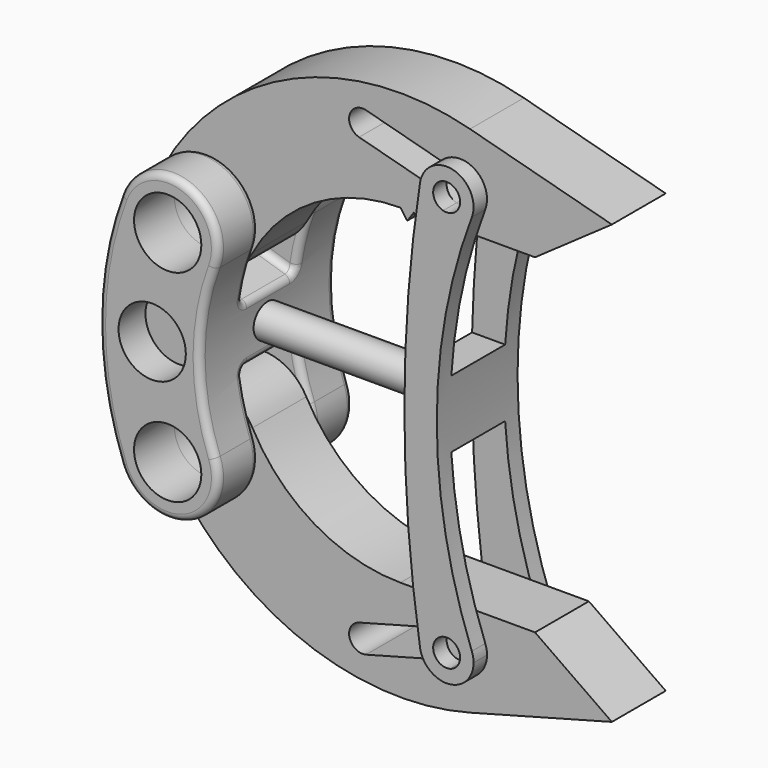
from build123d import *

# Parameters (mm, degrees)
F1_R           = 5
F2_DEPTH       = 5
F0_R           = 5
F3_DEPTH       = 12.5
F4_R           = 5
F5_DEPTH       = 25.001
F6_R           = 5
F7_DEPTH       = 5
F8_R           = 5
F9_DEPTH       = 7.5
F10_R          = 2.5
F11_DEPTH      = 10.2360656985
F11_DEPTH_BACK = 60.001
F12_R          = 2.5
F13_DEPTH      = 32
F13_DEPTH_BACK = 10
F15_DEPTH      = 7.5
F17_DEPTH      = 5
F18_R          = 1


with BuildPart() as f2:
    # F1 (on Front) → F2 (new body, symmetric)
    with BuildSketch(Plane.XZ):
        with BuildLine():
            ThreePointArc((38.9229935461, 38.1714845638), (12.7620087728, 36.2695311392), (-6.5959822677, 18.5697363943))
            ThreePointArc((-6.5959822677, 18.5697363943), (-3.5697363943, 8.4040177323), (6.5959822677, 11.4302636057))
            ThreePointArc((6.5959822677, 11.4302636057), (15.785676778, 21.0076181762), (28.5825898266, 24.5311422915))
            Line((28.5825898266, 24.5311422915), (30.5825898266, 24.5311422915))
            Line((30.5825898266, 24.5311422915), (32.5825898266, 24.5311422915))
            Line((32.5825898266, 24.5311422915), (48.5825898266, 24.5311422915))
            Line((48.5825898266, 24.5311422915), (60, 32.5311422915))
            Line((60, 32.5311422915), (38.9229935461, 38.1714845638))
        make_face()
        with Locations((0, 15)):
            Circle(F1_R, mode=Mode.SUBTRACT)
        with BuildLine():
            ThreePointArc((22.4425128865, 31.74578129), (21.0275159589, 34.1948185896), (23.4765532585, 35.6098155172))
            Line((23.4765532585, 35.6098155172), (37.9666816106, 31.7321641224))
            ThreePointArc((37.9666816106, 31.7321641224), (39.3816785382, 29.2831268228), (36.9326412386, 27.8681298951))
            Line((36.9326412386, 27.8681298951), (22.4425128865, 31.74578129))
        make_face(mode=Mode.SUBTRACT)
        Polygon((30.5825898266, 24.5311422915), (28.5825898266, 24.5311422915), (29.5949246287, 23.1395885348), align=None)
        Polygon((32.5825898266, 24.5311422915), (30.5825898266, 24.5311422915), (31.5949246287, 22.5311422915), align=None)
    extrude(amount=F2_DEPTH, both=True)


with BuildPart() as f2b:
    # F1 (on Front) → F2, piece 2 (new body, symmetric)
    with BuildSketch(Plane.XZ):
        with BuildLine():
            Line((38.9229935461, -38.1714845638), (60, -32.5311422915))
            Line((60, -32.5311422915), (48.5825898266, -24.5311422915))
            Line((48.5825898266, -24.5311422915), (28.5825898266, -24.5311422915))
            ThreePointArc((28.5825898266, -24.5311422915), (15.785676778, -21.0076181762), (6.5959822677, -11.4302636057))
            ThreePointArc((6.5959822677, -11.4302636057), (-3.5697363943, -8.4040177323), (-6.5959822677, -18.5697363943))
            ThreePointArc((-6.5959822677, -18.5697363943), (12.7620087728, -36.2695311392), (38.9229935461, -38.1714845638))
        make_face()
        with Locations((0, -15)):
            Circle(F1_R, mode=Mode.SUBTRACT)
        with BuildLine():
            Line((37.9666816106, -31.7321641224), (23.4765532585, -35.6098155172))
            ThreePointArc((23.4765532585, -35.6098155172), (21.0275159589, -34.1948185896), (22.4425128865, -31.74578129))
            Line((22.4425128865, -31.74578129), (36.9326412386, -27.8681298951))
            ThreePointArc((36.9326412386, -27.8681298951), (39.3816785382, -29.2831268228), (37.9666816106, -31.7321641224))
        make_face(mode=Mode.SUBTRACT)
    extrude(amount=F2_DEPTH, both=True)


with BuildPart() as f3:
    # F0 (on Front) → F3 (new body, symmetric)
    with BuildSketch(Plane.XZ):
        with BuildLine():
            ThreePointArc((7.0173413473, -12.3529411765), (4.7649343015, 0), (7.0173413473, 12.3529411765))
            ThreePointArc((7.0173413473, 12.3529411765), (2.6470588235, 22.0173413473), (-7.0173413473, 17.6470588235))
            ThreePointArc((-7.0173413473, 17.6470588235), (-10.2350656985, 0), (-7.0173413473, -17.6470588235))
            ThreePointArc((-7.0173413473, -17.6470588235), (2.6470588235, -22.0173413473), (7.0173413473, -12.3529411765))
        make_face()
        with Locations((0, -15)):
            Circle(F0_R, mode=Mode.SUBTRACT)
        with Locations((0, 15)):
            Circle(F0_R, mode=Mode.SUBTRACT)
    extrude(amount=F3_DEPTH, both=True)

    # F4 (on face) → F5 (cut, through all)
    with BuildSketch(Plane.XZ.offset(12.5)):
        with Locations((-2.3030399292, 0)):
            Circle(F4_R)
    extrude(amount=-F5_DEPTH, mode=Mode.SUBTRACT)

    # F6 (on Front) → F7 (cut, symmetric)
    with BuildSketch(Plane.XZ):
        with BuildLine():
            ThreePointArc((4.9936817324, 3.9949962177), (5.7478439471, 8.2363562222), (7.0173413473, 12.3529411765))
            ThreePointArc((7.0173413473, 12.3529411765), (2.6470588235, 22.0173413473), (-7.0173413473, 17.6470588235))
            ThreePointArc((-7.0173413473, 17.6470588235), (-8.4725761822, 13.1583654889), (-9.4981869819, 8.5524780864))
            Line((-9.4981869819, 8.5524780864), (4.9936817324, 3.9949962177))
        make_face()
        with Locations((0, 15)):
            Circle(F6_R, mode=Mode.SUBTRACT)
        with Locations((-2.3030399292, 0)):
            Circle(F6_R)
        with BuildLine():
            ThreePointArc((-9.4981869819, -8.5524780864), (-8.4725761822, -13.1583654889), (-7.0173413473, -17.6470588235))
            ThreePointArc((-7.0173413473, -17.6470588235), (2.6470588235, -22.0173413473), (7.0173413473, -12.3529411765))
            ThreePointArc((7.0173413473, -12.3529411765), (5.7478439471, -8.2363562222), (4.9936817324, -3.9949962177))
            Line((4.9936817324, -3.9949962177), (-9.4981869819, -8.5524780864))
        make_face()
        with Locations((0, -15)):
            Circle(F6_R, mode=Mode.SUBTRACT)
    extrude(amount=F7_DEPTH, both=True, mode=Mode.SUBTRACT)

    # F8 (on Front) → F9 (join, symmetric)
    with BuildSketch(Plane.XZ):
        with Locations((-2.3030399292, 0)):
            Circle(F8_R)
    extrude(amount=F9_DEPTH, both=True)

    # F10 (on Right) → F11 (cut, two sides)
    with BuildSketch(Plane.YZ) as f11_sk:
        Circle(F10_R)
    extrude(amount=-F11_DEPTH, mode=Mode.SUBTRACT)
    extrude(f11_sk.sketch, amount=F11_DEPTH_BACK, mode=Mode.SUBTRACT)

    # F18
    f18_edges = [f3.edges().sort_by_distance(p)[0] for p in [
        (4.764934, -12.5, 0),
        (4.764934, 12.5, 0),
        (4.993682, 0, -3.994996),
        (4.993682, 0, 3.994996),
        (-2.252253, 5, -6.273737),
        (-2.252253, 5, 6.273737),
        (-2.252253, -5, 6.273737),
        (-2.252253, -5, -6.273737),
        (2.647059, 12.5, 22.017341),
        (5.747844, 5, -8.236356),
        (5.747844, -5, -8.236356),
        (5.747844, 5, 8.236356),
        (5.747844, -5, 8.236356),
        (-8.472576, 5, 13.158365),
        (-10.235066, 12.5, 0),
        (-9.498187, 0, 8.552478),
        (-8.472576, 5, -13.158365),
        (-8.472576, -5, 13.158365),
        (-9.498187, 0, -8.552478),
        (-8.472576, -5, -13.158365),
        (-10.235066, -12.5, 0),
        (2.647059, 12.5, -22.017341),
        (2.647059, -12.5, -22.017341),
        (2.647059, -12.5, 22.017341),
    ]]
    fillet(f18_edges, radius=F18_R)


with BuildPart() as f13:
    # F12 (on Right) → F13 (new body, two sides)
    with BuildSketch(Plane.YZ) as f13_sk:
        Circle(F12_R)
    extrude(amount=F13_DEPTH)
    extrude(f13_sk.sketch, amount=-F13_DEPTH_BACK)

    # F14 (on Front) → F15 (join, symmetric)
    with BuildSketch(Plane.XZ):
        with BuildLine():
            ThreePointArc((41.1894854829, 28.3810923893), (41.3840798208, 29.0787928077), (41.4496614246, 29.8001470088))
            ThreePointArc((41.4496614246, 29.8001470088), (37.7546322392, 33.7885041646), (33.4961650235, 30.4083132742))
            ThreePointArc((33.4961650235, 30.4083132742), (36.4304361813, 25.9321785622), (41.1894854829, 28.3810923893))
        make_face()
        with BuildLine():
            ThreePointArc((39.4496614246, 29.8001470088), (38.6674380108, 28.2136350529), (36.9326412386, 27.8681298951))
            ThreePointArc((36.9326412386, 27.8681298951), (35.517644311, 30.3171671947), (37.9666816106, 31.7321641224))
            ThreePointArc((37.9666816106, 31.7321641224), (39.0361733804, 31.017923595), (39.4496614246, 29.8001470088))
        make_face(mode=Mode.SUBTRACT)
        with BuildLine():
            ThreePointArc((41.1894854829, 28.3810923893), (36.4304361813, 25.9321785622), (33.4961650235, 30.4083132742))
            ThreePointArc((33.4961650235, 30.4083132742), (31.1709850786, 0), (33.4961650235, -30.4083132742))
            ThreePointArc((33.4961650235, -30.4083132742), (36.4304361813, -25.9321785622), (41.1894854829, -28.3810923893))
            ThreePointArc((41.1894854829, -28.3810923893), (35.9859666487, 0), (41.1894854829, 28.3810923893))
        make_face()
        with BuildLine():
            ThreePointArc((41.1894854829, -28.3810923893), (36.4304361813, -25.9321785622), (33.4961650235, -30.4083132742))
            ThreePointArc((33.4961650235, -30.4083132742), (37.7546322392, -33.7885041646), (41.4496614246, -29.8001470088))
            ThreePointArc((41.4496614246, -29.8001470088), (41.3840798208, -29.0787928077), (41.1894854829, -28.3810923893))
        make_face()
        with BuildLine():
            ThreePointArc((37.9666816106, -31.7321641224), (35.517644311, -30.3171671947), (36.9326412386, -27.8681298951))
            ThreePointArc((36.9326412386, -27.8681298951), (38.6674380108, -28.2136350529), (39.4496614246, -29.8001470088))
            ThreePointArc((39.4496614246, -29.8001470088), (39.0361733804, -31.017923595), (37.9666816106, -31.7321641224))
        make_face(mode=Mode.SUBTRACT)
    extrude(amount=F15_DEPTH, both=True)

    # F16 (on Front) → F17 (cut, symmetric)
    with BuildSketch(Plane.XZ):
        with BuildLine():
            ThreePointArc((41.1894854829, 28.3810923893), (38.4688866679, 33.6681154553), (33.4961650235, 30.4083132742))
            ThreePointArc((33.4961650235, 30.4083132742), (31.9593315071, 17.7402672278), (31.2334948473, 5))
            Line((31.2334948473, 5), (36.1423695353, 5))
            ThreePointArc((36.1423695353, 5), (37.7871346697, 16.8802451737), (41.1894854829, 28.3810923893))
        make_face()
        with BuildLine():
            ThreePointArc((31.2334948473, -5), (31.9593315071, -17.7402672278), (33.4961650235, -30.4083132742))
            ThreePointArc((33.4961650235, -30.4083132742), (38.4688866679, -33.6681154553), (41.1894854829, -28.3810923893))
            ThreePointArc((41.1894854829, -28.3810923893), (37.7871346697, -16.8802451737), (36.1423695353, -5))
            Line((36.1423695353, -5), (31.2334948473, -5))
        make_face()
    extrude(amount=F17_DEPTH, both=True, mode=Mode.SUBTRACT)


solid = Compound([f2.part, f2b.part, f3.part, f13.part])
